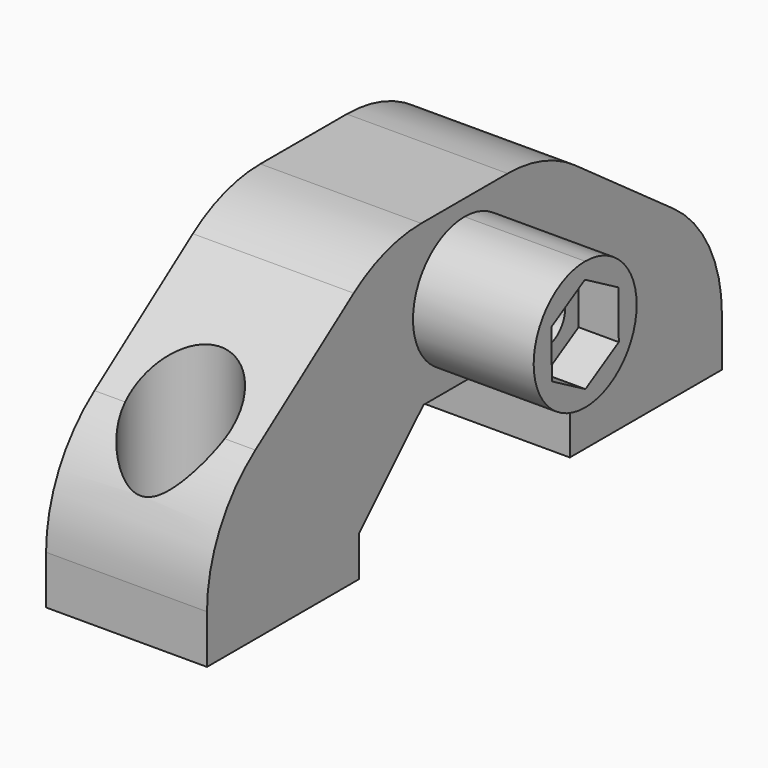
from build123d import *

# Parameters (mm, degrees)
F1_DEPTH       = 20
F3_DEPTH       = 15
F5_D           = 6.3
F5_DEPTH       = 30
F5_TIP         = 1.8927109499
F6_DEPTH       = 5
F8_D           = 6.6
F8_DEPTH       = 21
F8_START       = 18.1600674
F8_CBORE_D     = 12.5
F8_CBORE_DEPTH = 12
F8_TIP         = 1.9828400428
F9_T1_DEPTH    = 66.2237980807
F9_T3_DEPTH    = 48.9219521717
F10_SIZE       = 10


# Not quite as in the source:
# - a fillet or chamfer that OpenCascade refuses, or shapes differently, is made with other operations: its cross-section is extruded or revolved along the edge and cut away or added


with BuildPart() as f1:
    # F0 (on Right) → F1 (new body)
    with BuildSketch(Plane.YZ):
        Polygon((-16.375976861, 0), (-16.375976861, 10), (-16.375976861, 15), (16.375976861, 15), (16.375976861, 10), (16.375976861, 0), (40, 0), (40, 15.2900453504), (12.5, 35), (0, 35), (-12.5, 35), (-40, 15.2900453504), (-40, 0), align=None)
    extrude(amount=-F1_DEPTH)

    # F2 (on face) → F3 (join)
    with BuildSketch(Plane.YZ):
        with BuildLine():
            ThreePointArc((0, 17.0022554452), (5.6591519034, 19.3441438406), (8.0035544985, 25.0022546555))
            ThreePointArc((8.0035544985, 25.0022546555), (5.6591519034, 30.6603654705), (0, 33.0022538659))
            Line((0, 33.0022538659), (0, 17.0022554452))
        make_face()
        with BuildLine():
            Line((0, 17.0022554452), (0, 33.0022538659))
            ThreePointArc((0, 33.0022538659), (-7.9964455015, 25.0022546555), (0, 17.0022554452))
        make_face()
    extrude(amount=F3_DEPTH)

    # F5
    with Locations(Plane.YZ.offset(15)):
        with Locations((0.0035544985, 25.0022546555)):
            Hole(F5_D / 2, depth=F5_DEPTH)
            with Locations((0, 0, -(F5_DEPTH + F5_TIP / 2))):  # 118° drill point
                Cone(0, F5_D / 2, F5_TIP, mode=Mode.SUBTRACT)

    # F4 (on face) → F6 (cut)
    with BuildSketch(Plane.YZ.offset(15)):
        Polygon((5.1826206219, 28.040446128), (-0.0380634364, 31.0065532225), (-5.2171295598, 27.9683617501), (-5.1755116248, 21.9640631831), (0.0451724335, 18.9979560886), (5.2242385569, 22.036147561), align=None)
    extrude(amount=-F6_DEPTH, mode=Mode.SUBTRACT)

    # F8
    # its depths count from where the whole tool has entered the part; down to there all is cleared
    with Locations(Plane.XY.offset(35).offset(-F8_START)):
        with Locations((-10, 31.5875445392), (-10, -31.5875445392)):
            CounterBoreHole(F8_D / 2, F8_CBORE_D / 2, F8_CBORE_DEPTH, depth=F8_DEPTH)
            with Locations((0, 0, -(F8_DEPTH + F8_TIP / 2))):  # 118° drill point
                Cone(0, F8_D / 2, F8_TIP, mode=Mode.SUBTRACT)

    # F9: fillet of radius 18 on 4 edges, made by hand

    # F9_s2 → F9_t1 (cut)
    with BuildSketch(Plane.YZ.offset(-43.1118990403)):
        with BuildLine():
            ThreePointArc((40, 6.0452857343), (38.0116581667, 14.2688374458), (32.4859108054, 20.6755856144))
            Line((32.4859108054, 20.6755856144), (40, 15.2900453504))
            Line((40, 15.2900453504), (40, 6.0452857343))
        make_face()
        with BuildLine():
            ThreePointArc((-40, 6.0452857343), (-38.0116581667, 14.2688374458), (-32.4859108054, 20.6755856144))
            Line((-32.4859108054, 20.6755856144), (-40, 15.2900453504))
            Line((-40, 15.2900453504), (-40, 6.0452857343))
        make_face()
    extrude(amount=F9_T1_DEPTH, mode=Mode.SUBTRACT)

    # F9_s4 → F9_t3 (cut)
    with BuildSketch(Plane.YZ.offset(-34.4609760859)):
        with BuildLine():
            ThreePointArc((17.201520371, 31.6302998801), (12.2226324527, 34.1368812484), (6.7156095657, 35))
            Line((6.7156095657, 35), (12.5, 35))
            Line((12.5, 35), (17.201520371, 31.6302998801))
        make_face()
        with BuildLine():
            ThreePointArc((-6.7156095657, 35), (-12.2226324527, 34.1368812484), (-17.201520371, 31.6302998801))
            Line((-17.201520371, 31.6302998801), (-12.5, 35))
            Line((-12.5, 35), (-6.7156095657, 35))
        make_face()
    extrude(amount=F9_T3_DEPTH, mode=Mode.SUBTRACT)

    # F10
    f10_edges = [f1.edges().sort_by_distance(p)[0] for p in [
        (-10, 16.375977, 15),
        (-10, -16.375977, 15),
    ]]
    chamfer(f10_edges, length=F10_SIZE)


solid = f1.part
